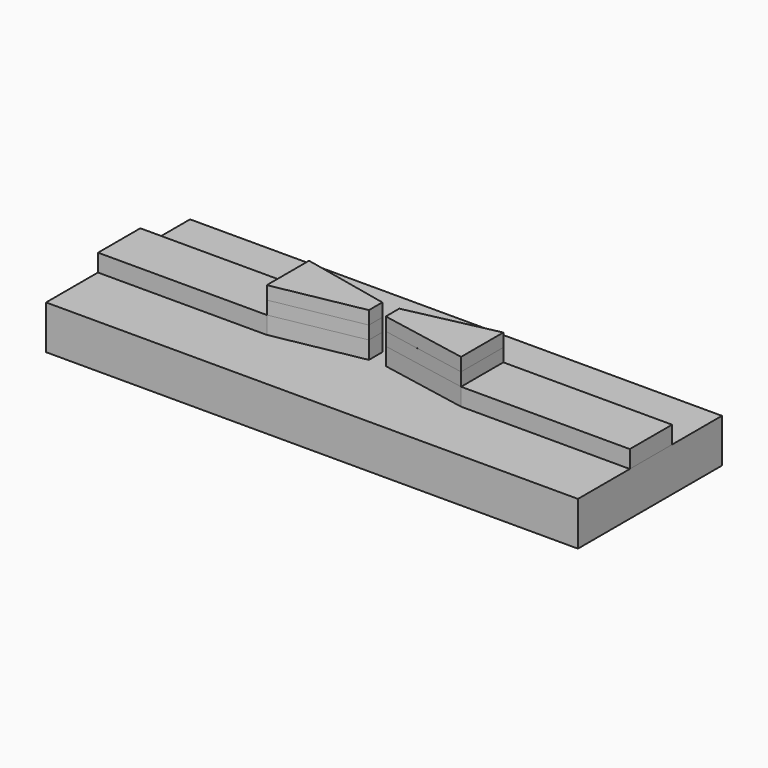
from build123d import *

# Parameters (mm, degrees)
F0_W     = 308.3111420274
F0_H     = 104.3191924691
F1_DEPTH = 25.4
F3_DEPTH = 10.16
F5_DEPTH = 7.62
F7_DEPTH = 7.62


# Not quite as in the source:
# - a feature names something its author has since deleted; it is built from what else it names


with BuildPart() as f1:
    # F0 (on Top) → F1 (new body)
    with BuildSketch(Plane.XY):
        with Locations((4.8579312861, 0)):
            Rectangle(F0_W, F0_H)
    extrude(amount=-F1_DEPTH)


with BuildPart() as f3:
    # F2 (on face) → F3 (new body)
    with BuildSketch(Plane.XY):
        Polygon((0, 4.8675285652), (-51.4132715762, 16.0222817212), (-149.2118090391, 16.0222817212), (-149.2118090391, -14.602586627), (-51.4132715762, -14.602586627), (0, -4.8675285652), align=None)
    extrude(amount=F3_DEPTH)


with BuildPart() as f3b:
    # F2 (on face) → F3, piece 2 (new body)
    with BuildSketch(Plane.XY):
        Polygon((159.022857435, 16.0222817212), (61.2243199721, 16.0222817212), (9.8110483959, 4.8675285652), (9.8110483959, -4.8675285652), (61.2243199721, -14.602586627), (159.022857435, -14.602586627), align=None)
    extrude(amount=F3_DEPTH)


with BuildPart() as f5:
    # F4 (on face) → F5 (new body)
    with BuildSketch(Plane.XY.offset(10.16)):
        Polygon((0, 4.8675285652), (-51.4132715762, 16.0222817212), (-51.4132715762, -14.602586627), (0, -4.8675285652), align=None)
    extrude(amount=F5_DEPTH)


with BuildPart() as f5b:
    # F4 (on face) → F5, piece 2 (new body)
    with BuildSketch(Plane.XY.offset(10.16)):
        Polygon((61.2102486193, 16.0119906068), (9.8198475316, 4.8690438271), (9.8198475316, -4.9016783014), (61.2102486193, -14.5960105583), align=None)
    extrude(amount=F5_DEPTH)


with BuildPart() as f7:
    # F6 (on face) → F7 (new body)
    with BuildSketch(Plane.XY.offset(17.78)):
        Polygon((0, 4.8675285652), (-51.4132715762, 16.0222817212), (-51.4132715762, -14.602586627), (0, -4.8675285652), align=None)
    extrude(amount=F7_DEPTH)


with BuildPart() as f7b:
    # F6 (on face) → F7, piece 2 (new body)
    with BuildSketch(Plane.XY.offset(17.78)):
        Polygon((61.2093545496, 16.0136017948), (9.8226387054, 4.8693544231), (9.8197283223, -4.9014249817), (61.2093545496, -14.5944608375), align=None)
    extrude(amount=F7_DEPTH)


solid = Compound([f1.part, f3.part, f3b.part, f5.part, f5b.part, f7.part, f7b.part])
